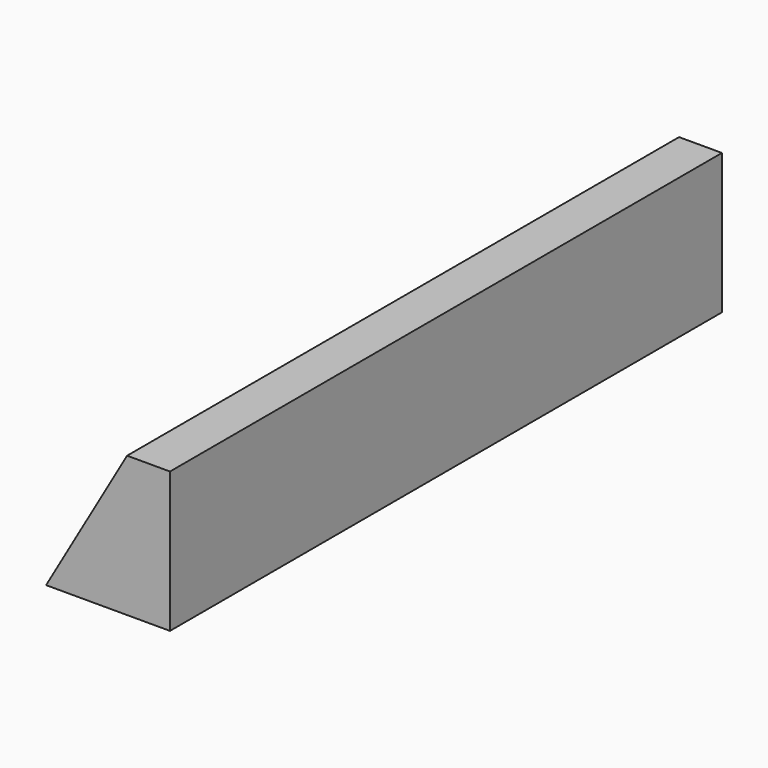
from build123d import *

# Parameters (mm, degrees)
F1_DEPTH = 44.25


with BuildPart() as f1:
    # F0 (on Front) → F1 (new body, symmetric)
    with BuildSketch(Plane.XZ):
        Polygon((-15.8923048454, 0), (0, 0), (0, 18), (-5.5, 18), align=None)
    extrude(amount=F1_DEPTH, both=True)


solid = f1.part
